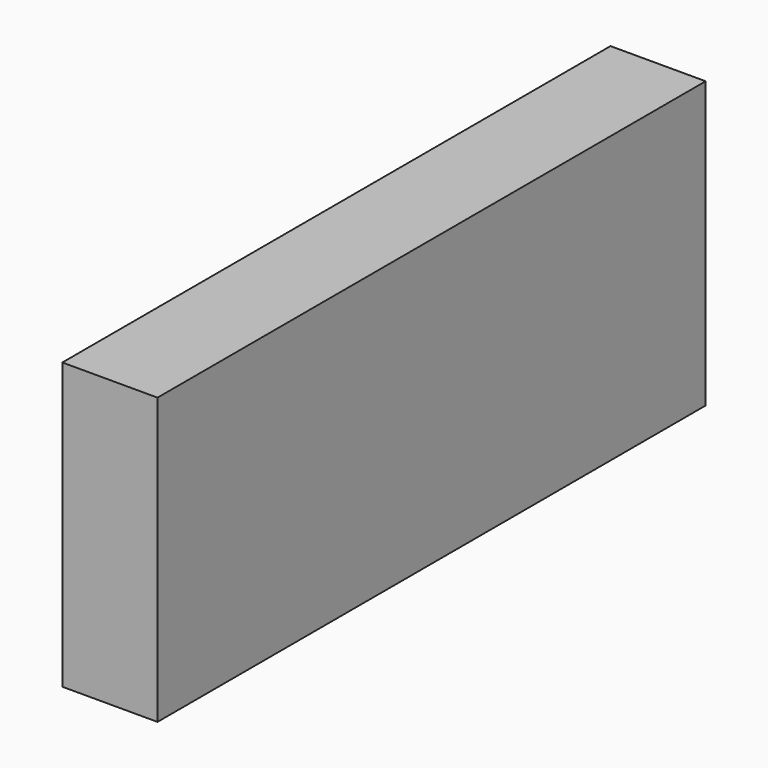
from build123d import *

# Parameters (mm, degrees)
F0_W     = 254
F0_H     = 762
F1_DEPTH = 1828.8
F2_W     = 25.4
F2_H     = 25.4
F3_DEPTH = 25.4
F4_R     = 16.4732072573
F5_DEPTH = 2.54


# Not quite as in the source:
# - a fillet or chamfer that OpenCascade refuses, or shapes differently, is made with other operations: its cross-section is extruded or revolved along the edge and cut away or added


with BuildPart() as f1:
    # F0 (on Front) → F1 (new body)
    with BuildSketch(Plane.XZ):
        Rectangle(F0_W, F0_H)
    extrude(amount=F1_DEPTH)

    # F2 (on face) → F3 (join)
    with BuildSketch(Plane(origin=(-127, 0, 0), x_dir=(0, -1, 0), z_dir=(-1, 0, 0))):
        with Locations((1689.1, 317.5)):
            Rectangle(F2_W, F2_H)
        with Locations((139.7, 317.5)):
            Rectangle(F2_W, F2_H)
    extrude(amount=F3_DEPTH)

    # F4 (on face) → F5 (join)
    with BuildSketch(Plane(origin=(-127, 0, 0), x_dir=(0, -1, 0), z_dir=(-1, 0, 0))):
        with Locations((1714.5154476166, 240.1719689369)):
            Circle(F4_R)
    extrude(amount=F5_DEPTH)

    # F6: fillet of radius 5.08 on 1 edges, made by hand

    # F6_s1 → F6_t2 (revolve, cut)
    with BuildSketch(Plane.XY.offset(240.1719689369)):
        with BuildLine():
            ThreePointArc((-127, -1730.9886548739), (-128.8594090512, -1729.1292458227), (-129.54, -1726.5892458227))
            Line((-129.54, -1726.5892458227), (-129.54, -1730.9886548739))
            Line((-129.54, -1730.9886548739), (-127, -1730.9886548739))
        make_face()
    revolve(axis=Axis((-129.54, -1714.5154476166, 240.1719689369), (-1, 0, 0)), mode=Mode.SUBTRACT)


solid = f1.part
